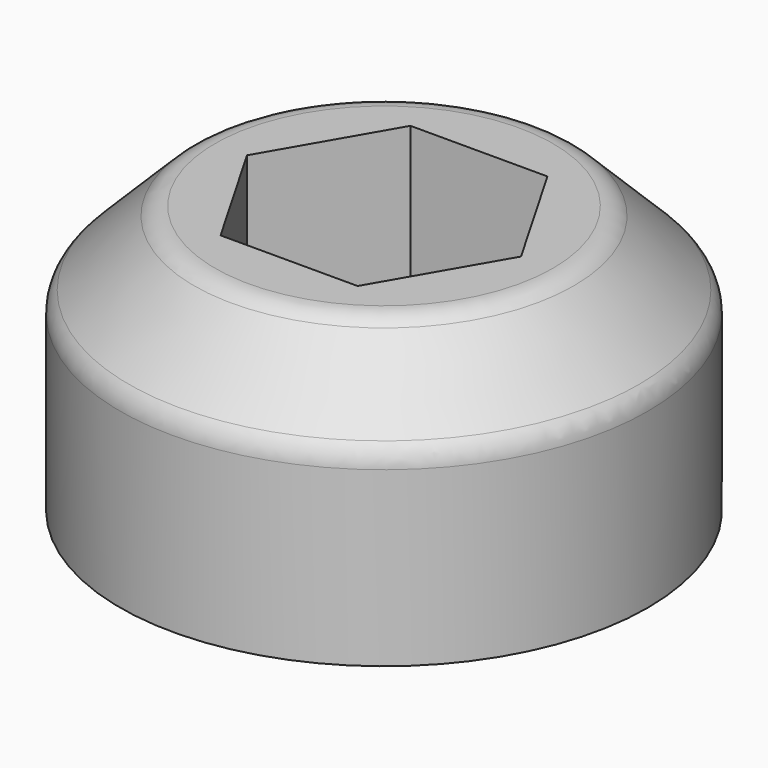
from build123d import *

# Parameters (mm, degrees)
F0_R     = 14.1859
F1_DEPTH = 14.4018
F2_SIZE  = 4.445
F3_R     = 1.5875


# Not quite as in the source:
# - a feature names something its author has since deleted; it is built from what else it names


with BuildPart() as f1:
    # F0 (on Top) → F1 (new body)
    with BuildSketch(Plane.XY):
        Circle(F0_R)
        Polygon((-7.366, 0), (-3.683, 6.3791431243), (3.683, 6.3791431243), (7.366, 0), (3.683, -6.3791431243), (-3.683, -6.3791431243), align=None, mode=Mode.SUBTRACT)
    extrude(amount=F1_DEPTH)

    # F2
    f2_edges = [f1.edges().sort_by_distance(p)[0] for p in [
        (-14.1859, 0, 14.4018),
    ]]
    chamfer(f2_edges, length=F2_SIZE)

    # F3
    f3_edges = [f1.edges().sort_by_distance(p)[0] for p in [
        (-9.7409, 0, 14.4018),
        (-14.1859, 0, 9.9568),
    ]]
    fillet(f3_edges, radius=F3_R)


solid = f1.part
